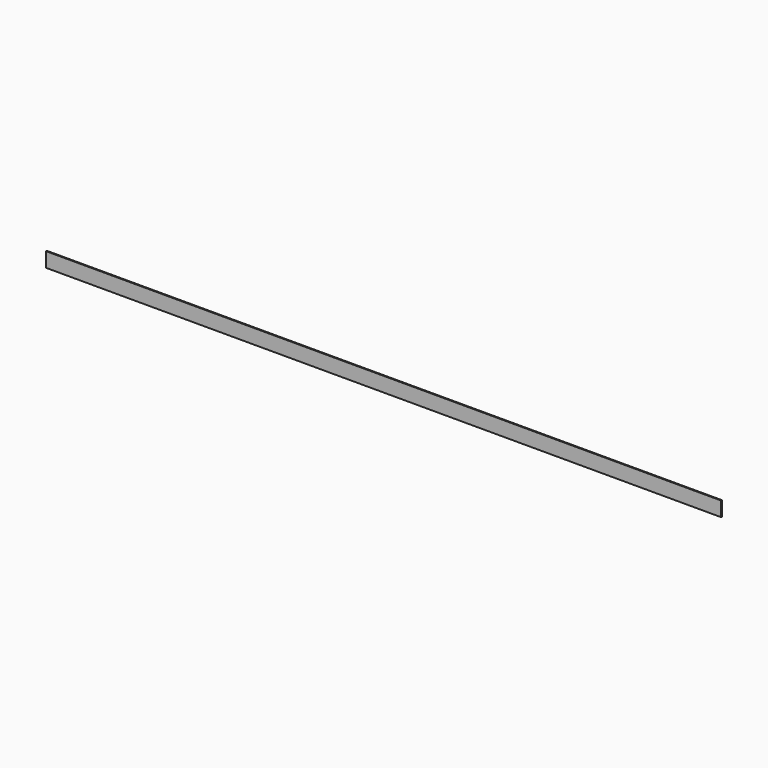
from build123d import *

# Parameters (mm, degrees)
F0_W     = 2336.8
F0_H     = 50.8
F1_DEPTH = 3.175


# Not quite as in the source:
# - a length typed as a fraction of an inch, garbled in the dataset ("3 / 203.2 mm" for 3/8 in), is restored


with BuildPart() as f1:
    # F0 (on Front) → F1 (new body)
    with BuildSketch(Plane.XZ):
        with Locations((710.5153441332, 12.1919997036)):
            Rectangle(F0_W, F0_H)
    extrude(amount=F1_DEPTH)


solid = f1.part
